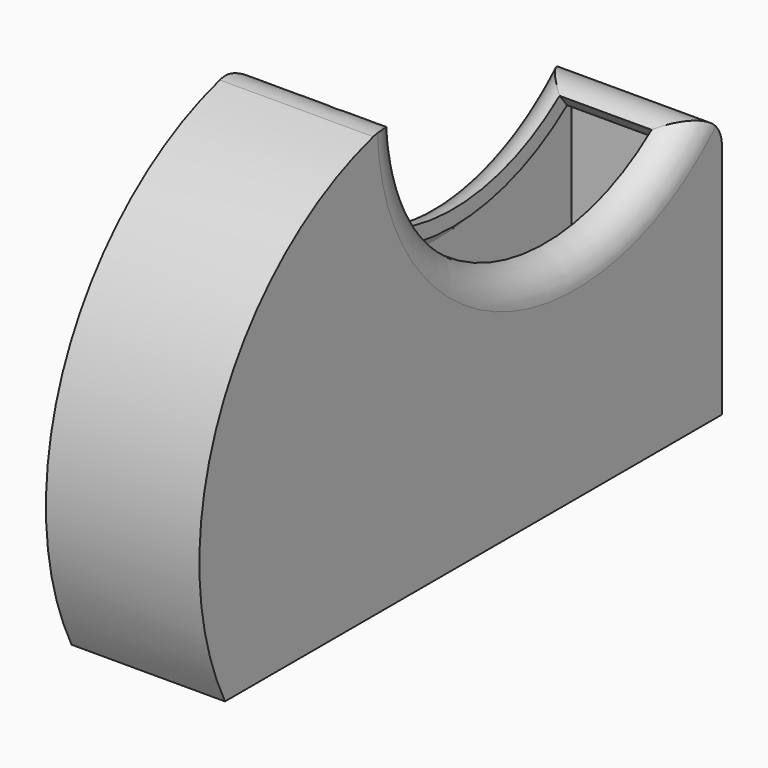
from build123d import *

# Parameters (mm, degrees)
F1_DEPTH = 25.4
F2_R     = 5.08
F3_T     = 2.54


# Not quite as in the source:
# - a shell that OpenCascade refuses in one call is made with other operations: the cavity is built on its own and cut out


with BuildPart() as f1:
    # F0 (on Right) → F1 (new body)
    with BuildSketch(Plane.YZ):
        with BuildLine():
            ThreePointArc((-6.8017239682, 18.9395658672), (-43.2327193048, -7.2897973695), (-43.3986243496, -52.1804355085))
            Line((-43.3986243496, -52.1804355085), (59.4223327935, -52.1804355085))
            Line((59.4223327935, -52.1804355085), (59.4223327935, 0))
            ThreePointArc((59.4223327935, 0), (19.2591298188, -15.1853432617), (-6.8017239682, 18.9395658672))
        make_face()
    extrude(amount=F1_DEPTH)

    # F2
    f2_edges = [f1.edges().sort_by_distance(p)[0] for p in [
        (12.7, 59.422333, 0),
        (12.7, -6.801724, 18.939566),
        (0, 19.25913, -15.185343),
        (25.4, 19.25913, -15.185343),
    ]]
    fillet(f2_edges, radius=F2_R)

    # F3: shell of thickness 2.54, made by hand


with BuildPart() as f3_core1:
    # F3_t2: copy of F1
    add(f1.part)

    # the walls: a layer under each face that stays
    f3_faces = [f3_core1.faces().sort_by_distance(p)[0] for p in [
        (12.7, 59.4223327935, -32.5906768925),
        (0, 5.3570087404, -17.1811267303),
        (12.7, 56.5735474159, -8.4371389974),
        (12.7, 8.0118542219, -52.1804355085),
        (25.4, 5.3570087404, -17.1811267303),
        (1.4878975516, 15.4764567571, -15.4748956916),
        (12.7, -44.5374630823, -10.0289336824),
        (12.7, -8.6201931506, 17.0491329967),
        (23.9121024484, 15.4766540031, -15.4749730413),
    ]]
    thicken(f3_faces, amount=-F3_T, mode=Mode.SUBTRACT)


with BuildPart() as f1_1:
    add(f1.part)

    # what is left inside the walls is the cavity
    f3_cavity = [f3_core1.part.solids().sort_by_distance(p)[0] for p in [
        (22.8346, 5.357009, -27.999693),
    ]]
    add(f3_cavity, mode=Mode.SUBTRACT)


solid = f1_1.part
